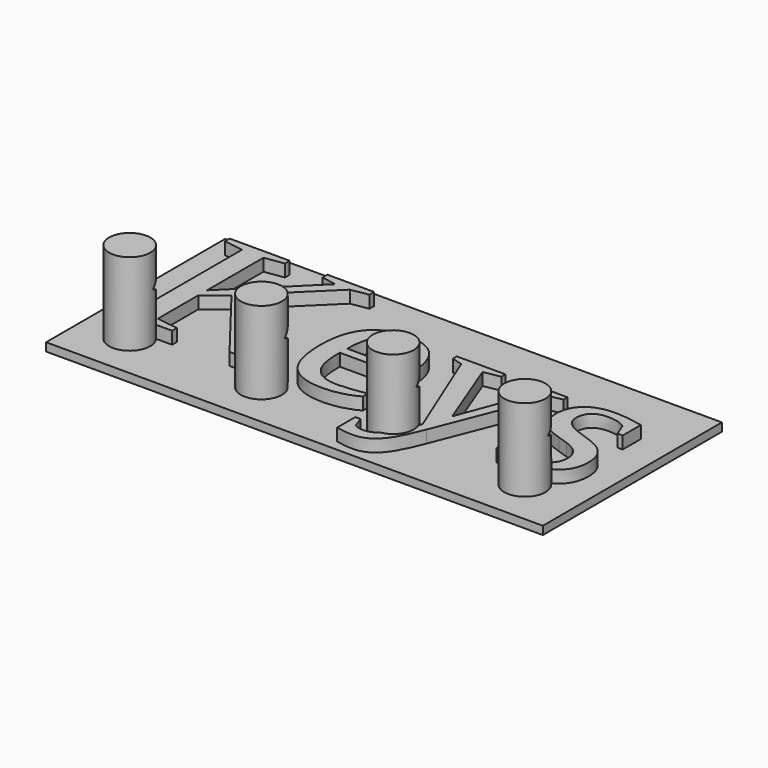
from build123d import *

# Parameters (mm, degrees)
F2_W          = 153.2573029399
F2_H          = 69.0584871918
F3_DEPTH      = 2.54
F0_TEXT_SIZE  = 70.5555555556
F4_DEPTH      = 3.81
F1_R          = 6.35
F5_DEPTH      = 25.4
F7_DEPTH      = 76.7471882042
F7_DEPTH_BACK = 76.5121149357


# Not quite as in the source:
# - Text() gives the source's letters only with a copy of the font that has no kerning and outlines rounded to 1/6400 em; it was checked with that copy


with BuildPart() as f3:
    # F2 (on Top) → F3 (new body)
    with BuildSketch(Plane.XY):
        with Locations((-0.1175366342, 16.5870105848)):
            Rectangle(F2_W, F2_H)
    extrude(amount=-F3_DEPTH)

    # F0 (on Top) → F4 (join)
    with BuildSketch(Plane.XY):
        with Locations((-73.4328993056, 0)):
            Text('Keys', F0_TEXT_SIZE, font='Tinos', text_align=(TextAlign.LEFT, TextAlign.BOTTOM))
    extrude(amount=F4_DEPTH)

    # F1 (on Top) → F5 (join)
    with BuildSketch(Plane.XY):
        with Locations((59.7219198775, -3.8784022909)):
            Circle(F1_R)
        with Locations((-21.5580801225, -3.8784022909)):
            Circle(F1_R)
        with Locations((19.0819198775, -3.8784022909)):
            Circle(F1_R)
        with Locations((-62.1980801225, -3.8784022909)):
            Circle(F1_R)
    extrude(amount=F5_DEPTH)

    # F6 (on Right) → F7 (cut, two sides)
    with BuildSketch(Plane.YZ) as f7_sk:
        Polygon((5.0294972025, 19.3757954985), (-2.7226332705, 14.9001008831), (5.0294972025, 10.4244062677), align=None)
    extrude(amount=-F7_DEPTH, mode=Mode.SUBTRACT)
    extrude(f7_sk.sketch, amount=F7_DEPTH_BACK, mode=Mode.SUBTRACT)


solid = f3.part
